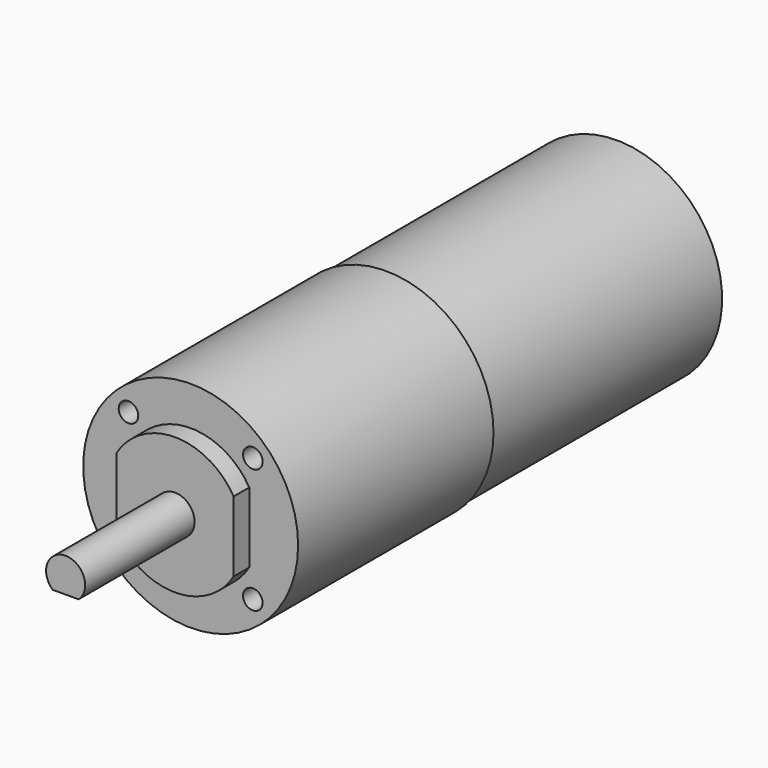
from build123d import *

# Parameters (mm, degrees)
F0_R      = 11
F1_DEPTH  = 25
F2_R      = 10.8
F3_DEPTH  = 29.5
F5_DEPTH  = 2
F6_R      = 2
F7_DEPTH  = 14
F9_DEPTH  = 8
F10_SIZE  = 0.49999
F11_R     = 1
F12_DEPTH = 3


# Not quite as in the source:
# - a fillet or chamfer is up to 0.001 mm smaller than in the source, because OpenCascade refuses the exact size


with BuildPart() as f1:
    # F0 (on Front) → F1 (new body)
    with BuildSketch(Plane.XZ):
        Circle(F0_R)
    extrude(amount=-F1_DEPTH)

    # F2 (on face) → F3 (join)
    with BuildSketch(Plane(origin=(0, 25, 0), x_dir=(-1, 0, 0), z_dir=(0, 1, 0))):
        Circle(F2_R)
    extrude(amount=F3_DEPTH)

    # F4 (on face) → F5 (join)
    with BuildSketch(Plane.XZ):
        with BuildLine():
            Line((6, -3.6055512755), (6, 3.6055512755))
            ThreePointArc((6, 3.6055512755), (0, 7), (-6, 3.6055512755))
            Line((-6, 3.6055512755), (-6, -3.6055512755))
            ThreePointArc((-6, -3.6055512755), (0, -7), (6, -3.6055512755))
        make_face()
    extrude(amount=F5_DEPTH)

    # F6 (on face) → F7 (join)
    with BuildSketch(Plane.XZ.offset(2)):
        Circle(F6_R)
    extrude(amount=F7_DEPTH)

    # F8 (on face) → F9 (cut)
    with BuildSketch(Plane.XZ.offset(16)):
        with BuildLine():
            ThreePointArc((-1.3228756555, -1.5), (0, -2), (1.3228756555, -1.5))
            Line((1.3228756555, -1.5), (-1.3228756555, -1.5))
        make_face()
    extrude(amount=-F9_DEPTH, mode=Mode.SUBTRACT)

    # F10 (size 0.5 in the source; OpenCascade refuses exactly that, so slightly less here)
    f10_edges = [f1.edges().sort_by_distance(p)[0] for p in [
        (0, -8, -1.5),
    ]]
    chamfer(f10_edges, length=F10_SIZE)

    # F11 (on face) → F12 (cut)
    with BuildSketch(Plane.XZ):
        with Locations((6.3639610307, -6.3639610307)):
            Circle(F11_R)
        with Locations((-6.3639610307, -6.3639610307)):
            Circle(F11_R)
        with Locations((-6.3639610307, 6.3639610307)):
            Circle(F11_R)
        with Locations((6.3639610307, 6.3639610307)):
            Circle(F11_R)
    extrude(amount=-F12_DEPTH, mode=Mode.SUBTRACT)


solid = f1.part
